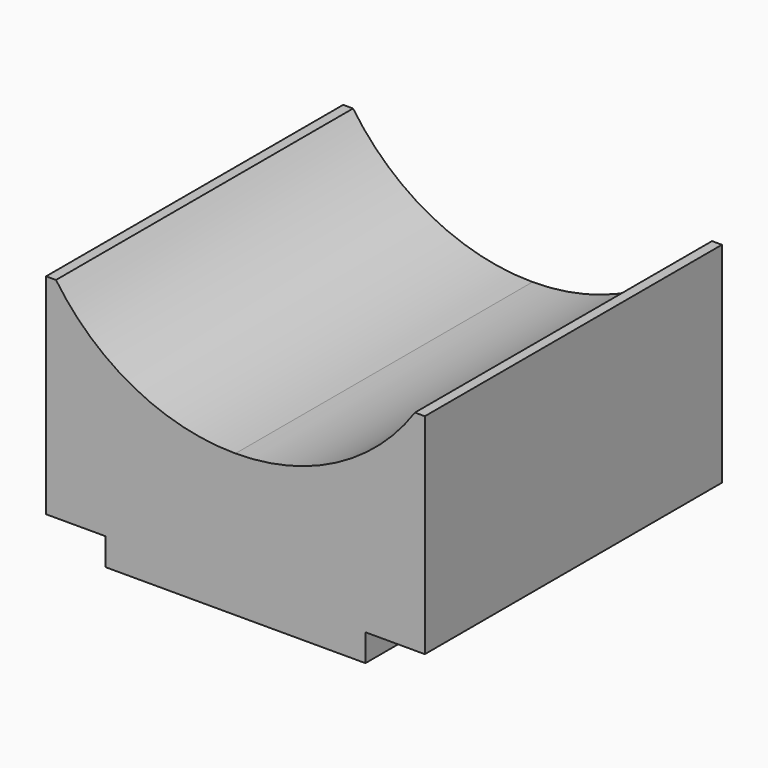
from build123d import *

# Parameters (mm, degrees)
F1_DEPTH = 15


# Not quite as in the source:
# - ends of sketch curves that miss each other by under 0.0002 mm in the source are joined


with BuildPart() as f1:
    # F0 (on Front) → F1 (new body)
    with BuildSketch(Plane.XZ):
        with BuildLine():
            Line((7.65, 4.781237), (7.250144, 4.781237))
            ThreePointArc((7.250144, 4.781237), (4.0957152155, 1.9799825245), (0, 0.968764))
            ThreePointArc((0, 0.968764), (-4.0957149647, 1.9799823926), (-7.2501430423, 4.7812369709))
            Line((-7.2501430423, 4.7812369709), (-7.65, 4.781237))
            Line((-7.65, 4.781237), (-7.65, -3.681236))
            Line((-7.65, -3.681236), (-5.25, -3.681236))
            Line((-5.25, -3.681236), (-5.25, -4.781236))
            Line((-5.25, -4.781236), (0, -4.781236))
            Line((0, -4.781236), (5.25, -4.781236))
            Line((5.25, -4.781236), (5.25, -3.681236))
            Line((5.25, -3.681236), (7.65, -3.681236))
            Line((7.65, -3.681236), (7.65, 4.781237))
        make_face()
    extrude(amount=F1_DEPTH)


solid = f1.part
